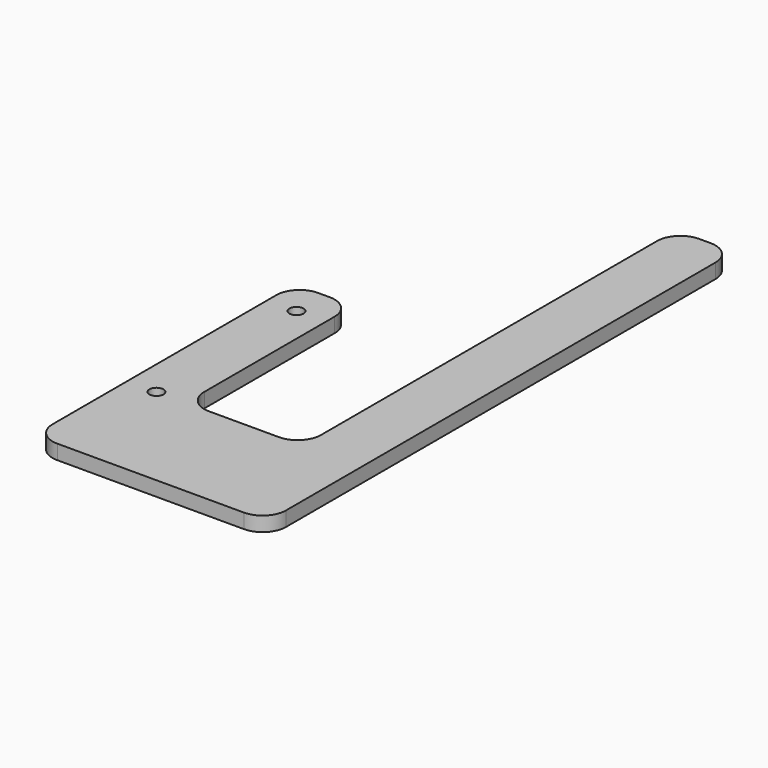
from build123d import *

# Parameters (mm, degrees)
F0_R     = 1.524
F0_W     = 12.7
F0_H     = 25.4
F1_DEPTH = 3.175
F2_R     = 5.08


with BuildPart() as f1:
    # F0 (on Top) → F1 (new body)
    with BuildSketch(Plane.XY):
        Polygon((1.1870916933, -2.6605168543), (-24.2129083067, -2.6605168543), (-24.2129083067, 42.9525971413), (-36.9129083067, 42.9525971413), (-36.9129083067, -2.6605168543), (-36.9129083067, -12.0184096301), (-36.9129083067, -28.0605168543), (13.8870916933, -28.0605168543), (13.8870916933, -12.0184096301), (13.8870916933, -2.6605168543), (13.8870916933, 73.5394831457), (1.1870916933, 73.5394831457), align=None)
        with Locations((-30.5629083067, -2.6605168543)):
            Circle(F0_R, mode=Mode.SUBTRACT)
        with Locations((-30.5629083067, 35.4394831457)):
            Circle(F0_R, mode=Mode.SUBTRACT)
        with Locations((7.5370916933, 86.2394831457)):
            Rectangle(F0_W, F0_H)
    extrude(amount=F1_DEPTH)

    # F2
    f2_edges = [f1.edges().sort_by_distance(p)[0] for p in [
        (-36.912908, 42.952597, 1.5875),
        (1.187092, -2.660517, 1.5875),
        (-36.912908, -28.060517, 1.5875),
        (13.887092, -28.060517, 1.5875),
        (-24.212908, -2.660517, 1.5875),
        (1.187092, 98.939483, 1.5875),
        (13.887092, 98.939483, 1.5875),
        (-24.212908, 42.952597, 1.5875),
    ]]
    fillet(f2_edges, radius=F2_R)


solid = f1.part
